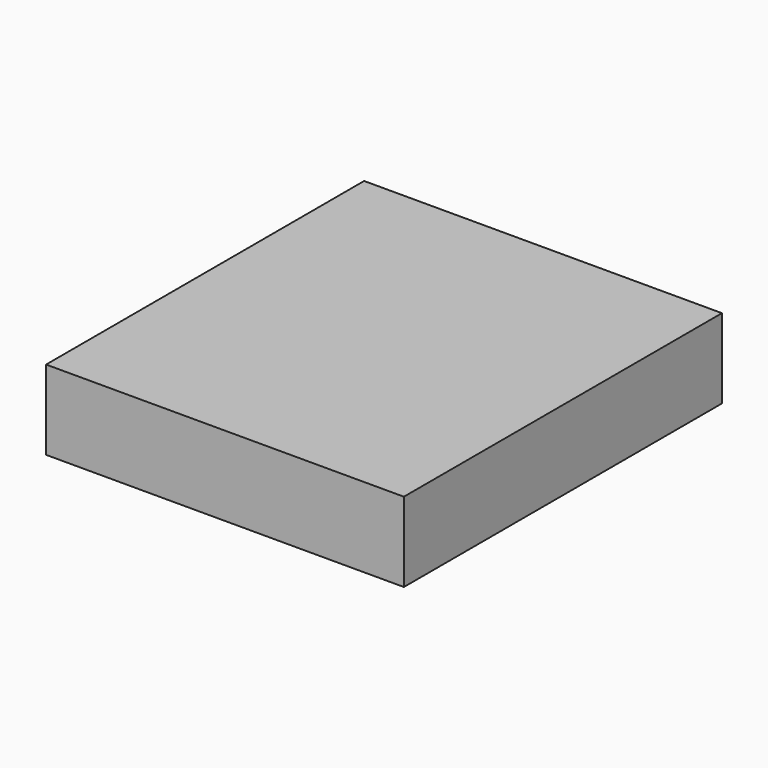
from build123d import *

# Parameters (mm, degrees)
F0_W     = 1800
F0_H     = 2000
F1_DEPTH = 400


# Not quite as in the source:
# - the program builds the solid bodies; features that only make, move or delete a surface that nothing else refers to are left out


with BuildPart() as f1:
    # F0 (on Top) → F1 (new body)
    with BuildSketch(Plane.XY):
        with Locations((900, 1000)):
            Rectangle(F0_W, F0_H)
    extrude(amount=F1_DEPTH)


solid = f1.part
